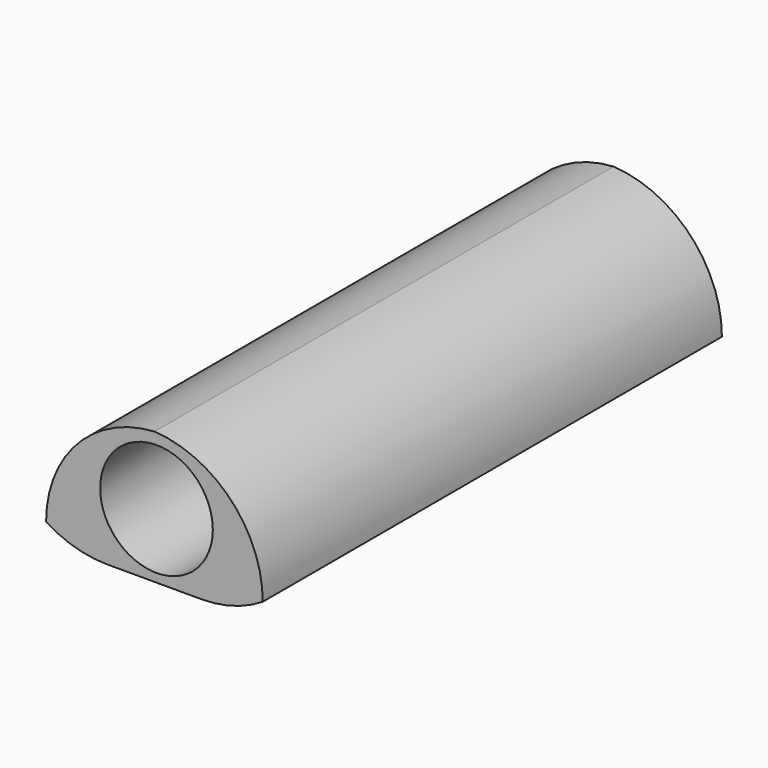
from build123d import *

# Parameters (mm, degrees)
F0_W        = 47.9449257255
F0_H        = 29.3166413903
F1_DEPTH    = 127
F3_R        = 12.4646622314
F4_DEPTH    = 127
F5_T1_DEPTH = 254
F6_T1_DEPTH = 194.7542070367
F7_T1_DEPTH = 194.7542070365


# Not quite as in the source:
# - a fillet or chamfer that OpenCascade refuses, or shapes differently, is made with other operations: its cross-section is extruded or revolved along the edge and cut away or added


with BuildPart() as f1:
    # F0 (on Front) → F1 (new body)
    with BuildSketch(Plane.XZ):
        with Locations((-23.9724628627, 14.6583206952)):
            Rectangle(F0_W, F0_H)
    extrude(amount=F1_DEPTH)

    # F3 (on face) → F4 (cut)
    with BuildSketch(Plane.XZ.offset(127)):
        with Locations((-23.5143899918, 14.3529390916)):
            Circle(F3_R)
    extrude(amount=-F4_DEPTH, mode=Mode.SUBTRACT)

    # F5: fillet of radius 25.4 on 2 edges, made by hand

    # F5_s2 → F5_t1 (cut)
    with BuildSketch(Plane.XZ.offset(-63.5)):
        with BuildLine():
            ThreePointArc((-47.9449257255, 3.9166413903), (-40.5054379676, 21.8771536325), (-22.5449257255, 29.3166413903))
            Line((-22.5449257255, 29.3166413903), (-47.9449257255, 29.3166413903))
            Line((-47.9449257255, 29.3166413903), (-47.9449257255, 3.9166413903))
        make_face()
        with BuildLine():
            ThreePointArc((0, 3.9166413903), (-7.4394877579, 21.8771536325), (-25.4, 29.3166413903))
            Line((-25.4, 29.3166413903), (0, 29.3166413903))
            Line((0, 29.3166413903), (0, 3.9166413903))
        make_face()
    extrude(amount=F5_T1_DEPTH, mode=Mode.SUBTRACT)

    # F6: fillet of radius 25.4 on 1 edges, made by hand

    # F6_s2 → F6_t1 (cut)
    with BuildSketch(Plane.XZ.offset(-33.8771035184)):
        with BuildLine():
            ThreePointArc((-13.5508414073, 0), (-6.4980869343, 0.9987980963), (0, 3.9166413903))
            Line((0, 3.9166413903), (0, 0))
            Line((0, 0), (-13.5508414073, 0))
        make_face()
    extrude(amount=F6_T1_DEPTH, mode=Mode.SUBTRACT)

    # F7: fillet of radius 25.4 on 1 edges, made by hand

    # F7_s2 → F7_t1 (cut)
    with BuildSketch(Plane.XZ.offset(-33.8771035183)):
        with BuildLine():
            ThreePointArc((-34.3940843182, 0), (-41.4468387912, 0.9987980963), (-47.9449257255, 3.9166413903))
            Line((-47.9449257255, 3.9166413903), (-47.9449257255, 0))
            Line((-47.9449257255, 0), (-34.3940843182, 0))
        make_face()
    extrude(amount=F7_T1_DEPTH, mode=Mode.SUBTRACT)


solid = f1.part
